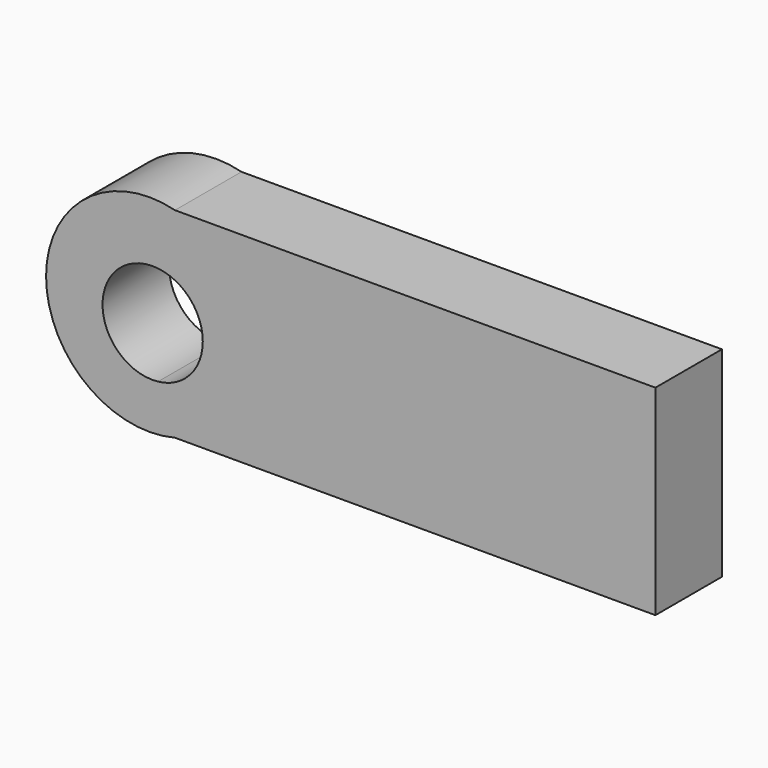
from build123d import *

# Parameters (mm, degrees)
F1_DEPTH = 25.4
F3_DEPTH = 25.4


# Not quite as in the source:
# - a feature names something its author has since deleted; it is built from what else it names


with BuildPart() as f1:
    # F0 (on Front) → F1 (new body)
    with BuildSketch(Plane.XZ):
        with BuildLine():
            Line((75.9890973568, -30.600361526), (75.9890973568, 30.600361526))
            Line((75.9890973568, 30.600361526), (-70.8035532623, 30.600361526))
            ThreePointArc((-70.8035532623, 30.600361526), (-53.6695268316, 19.3760533103), (-47.026597149, 0))
            ThreePointArc((-47.026597149, 0), (-53.6695268316, -19.3760533103), (-70.8035532623, -30.600361526))
            Line((-70.8035532623, -30.600361526), (75.9890973568, -30.600361526))
        make_face()
    extrude(amount=F1_DEPTH)

    # F0 (on Front) → F3 (join)
    with BuildSketch(Plane.XZ):
        with BuildLine():
            Line((75.9890973568, -30.600361526), (75.9890973568, 30.600361526))
            Line((75.9890973568, 30.600361526), (-70.8035532623, 30.600361526))
            ThreePointArc((-70.8035532623, 30.600361526), (-53.6695268316, 19.3760533103), (-47.026597149, 0))
            ThreePointArc((-47.026597149, 0), (-53.6695268316, -19.3760533103), (-70.8035532623, -30.600361526))
            Line((-70.8035532623, -30.600361526), (75.9890973568, -30.600361526))
        make_face()
        with BuildLine():
            ThreePointArc((-47.026597149, 0), (-53.6695268316, 19.3760533103), (-70.8035532623, 30.600361526))
            Line((-70.8035532623, 30.600361526), (-75.9890973568, 30.600361526))
            Line((-75.9890973568, 30.600361526), (-75.9890973568, 13.2593563534))
            ThreePointArc((-75.9890973568, 13.2593563534), (-66.2306105471, 8.26762835), (-62.3079244328, -1.9675046206))
            ThreePointArc((-62.3079244328, -1.9675046206), (-66.2306105471, -12.2026375911), (-75.9890973568, -17.1943655945))
            Line((-75.9890973568, -17.1943655945), (-75.9890973568, -30.600361526))
            Line((-75.9890973568, -30.600361526), (-70.8035532623, -30.600361526))
            ThreePointArc((-70.8035532623, -30.600361526), (-53.6695268316, -19.3760533103), (-47.026597149, 0))
        make_face()
        with BuildLine():
            Line((-75.9890973568, 30.600361526), (-70.8035532623, 30.600361526))
            ThreePointArc((-70.8035532623, 30.600361526), (-110.1854708241, 0), (-70.8035532623, -30.600361526))
            Line((-70.8035532623, -30.600361526), (-75.9890973568, -30.600361526))
            Line((-75.9890973568, -30.600361526), (-75.9890973568, -17.1943655945))
            ThreePointArc((-75.9890973568, -17.1943655945), (-92.9362769889, -1.9675046206), (-75.9890973568, 13.2593563534))
            Line((-75.9890973568, 13.2593563534), (-75.9890973568, 30.600361526))
        make_face()
    extrude(amount=F3_DEPTH)


solid = f1.part
